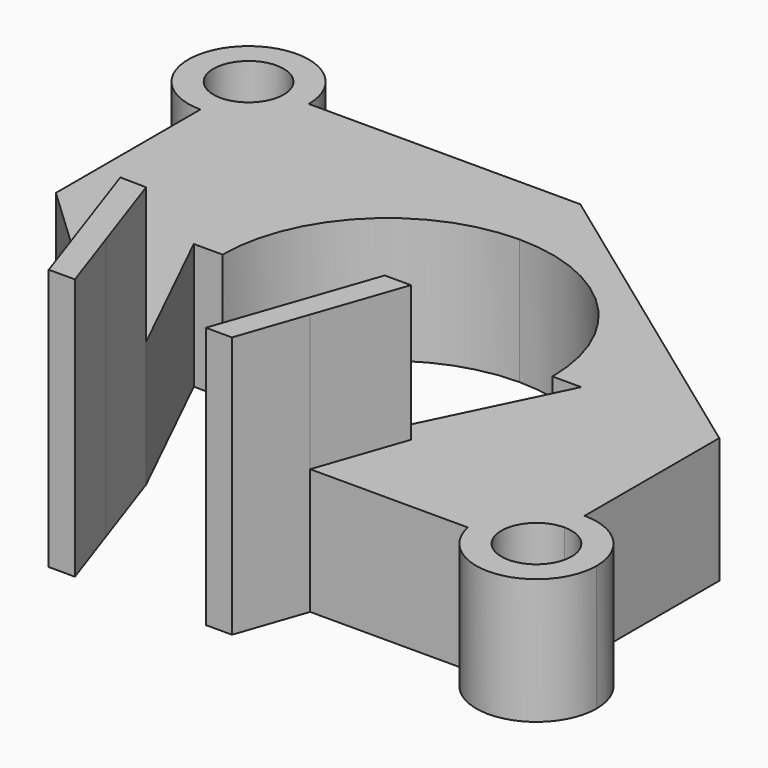
from build123d import *

# Parameters (mm, degrees)
F1_DEPTH = 12
F2_DEPTH = 25


# Not quite as in the source:
# - ends of sketch curves that miss each other by under 0.0002 mm in the source are joined


with BuildPart() as f1:
    # F0 (on Top) → F1 (new body)
    with BuildSketch(Plane.XY):
        with BuildLine():
            ThreePointArc((-55.8174114415, 34.8348648238), (-58.1862191586, 40.5536725408), (-52.4674114416, 38.1848648238))
            Line((-52.4674114416, 38.1848648238), (-50.0674114416, 38.1848649627))
            ThreePointArc((-50.0674114416, 38.1848649627), (-59.8832754334, 42.2507288156), (-55.8174114415, 32.4348648238))
            Line((-55.8174114415, 32.4348648238), (-55.8174114415, 34.8348648238))
        make_face()
        with BuildLine():
            Line((-50.0674114416, 38.1848649627), (-52.4674114416, 38.1848649047))
            ThreePointArc((-52.4674114416, 38.1848649047), (-53.4486037246, 35.8160571069), (-55.8174114415, 34.8348648238))
            Line((-55.8174114415, 34.8348648238), (-55.8174114415, 32.4348648238))
            ThreePointArc((-55.8174114415, 32.4348648238), (-51.7515474497, 34.119000832), (-50.0674114416, 38.1848649627))
        make_face()
        with BuildLine():
            Line((-24.1338443596, 38.184865589), (-50.0674114416, 38.1848649627))
            ThreePointArc((-50.0674114416, 38.1848649627), (-51.7515474497, 34.119000832), (-55.8174114415, 32.4348648238))
            Line((-55.8174114415, 32.4348648238), (-55.8174114412, 15.1848640586))
            Line((-55.8174114412, 15.1848640586), (-42.6338443592, 15.1659585535))
            ThreePointArc((-42.6338443592, 15.1659585535), (-37.2153198113, 28.2474340054), (-24.1338443595, 33.6659585535))
            Line((-24.1338443595, 33.6659585535), (-24.1338443596, 38.184865589))
        make_face()
        with BuildLine():
            Line((-24.1338443595, 30.9159585535), (-24.1338443595, 33.6659585535))
            ThreePointArc((-24.1338443595, 33.6659585535), (-37.2153198113, 28.2474340054), (-42.6338443592, 15.1659585535))
            Line((-42.6338443592, 15.1659585535), (-39.8838443592, 15.1659585535))
            ThreePointArc((-39.8838443592, 15.1659585535), (-35.270776163, 26.3028903571), (-24.1338443595, 30.9159585535))
        make_face()
        with BuildLine():
            Line((7.5497227227, 15.1659585535), (-24.1338443596, 38.184865589))
            Line((-24.1338443596, 38.184865589), (-24.1338443595, 33.6659585535))
            ThreePointArc((-24.1338443595, 33.6659585535), (-11.0523689074, 28.2474340056), (-5.6338443592, 15.1659585535))
            Line((-5.6338443592, 15.1659585535), (7.5497227227, 15.1659585535))
        make_face()
        with BuildLine():
            ThreePointArc((-5.6338443592, 15.1659585535), (-11.0523689074, 28.2474340056), (-24.1338443595, 33.6659585535))
            Line((-24.1338443595, 33.6659585535), (-24.1338443595, 30.9159585535))
            ThreePointArc((-24.1338443595, 30.9159585535), (-12.9969125556, 26.3028903573), (-8.3838443592, 15.1659585535))
            Line((-8.3838443592, 15.1659585535), (-5.6338443592, 15.1659585535))
        make_face()
        with BuildLine():
            Line((7.549722723, -0.909568585), (7.5497227227, 15.1659585535))
            Line((7.5497227227, 15.1659585535), (-5.6338443592, 15.1659585535))
            Line((-5.6338443592, 15.1659585535), (-12.7387191109, 0.5919707473))
            Line((-12.7387191109, 0.5919707473), (-10.2387191109, 0.5919707473))
            Line((-10.2387191109, 0.5919707473), (-13.136122196, -7.8151351762))
            Line((-13.136122196, -7.8151351762), (1.9170354556, -7.8151351762))
            ThreePointArc((1.9170354556, -7.8151351762), (3.0939956275, -3.0251503303), (7.549722723, -0.909568585))
        make_face()
        Polygon((-42.6338443592, 15.1659585535), (-55.8174114412, 15.1848640586), (-36.8837256357, -2.690086035), (-38.0284454354, 0.643162408), (-35.5289696075, 0.5919707473), align=None)
        with BuildLine():
            ThreePointArc((13.2997227231, -6.659568585), (11.6155867149, -2.5937045931), (7.549722723, -0.909568585))
            ThreePointArc((7.549722723, -0.909568585), (3.0939956275, -3.0251503303), (1.9170354556, -7.8151351762))
            ThreePointArc((1.9170354556, -7.8151351762), (8.1304757738, -12.3801652229), (13.2997227231, -6.659568585))
        make_face()
        with BuildLine():
            ThreePointArc((10.8997227231, -6.659568585), (5.1809150061, -9.028376302), (7.549722723, -3.309568585))
            ThreePointArc((7.549722723, -3.309568585), (9.91853044, -4.290760868), (10.8997227231, -6.659568585))
        make_face(mode=Mode.SUBTRACT)
        Polygon((-38.0284454354, 0.643162408), (-36.8837256357, -2.690086035), (-35.1236572441, -7.8151351762), (-32.6315665225, -7.8151351762), (-35.5289696075, 0.5919707473), align=None)
        Polygon((-32.6315665225, -7.8151351762), (-35.1236572441, -7.8151351762), (-32.8838443592, -14.3371266833), (-30.3838443592, -14.3371266833), align=None)
        Polygon((-13.136122196, -7.8151351762), (-15.636122196, -7.8151351762), (-17.8838443592, -14.3371266833), (-15.3838443592, -14.3371266833), align=None)
        Polygon((-10.2387191109, 0.5919707473), (-12.7387191109, 0.5919707473), (-15.636122196, -7.8151351762), (-13.136122196, -7.8151351762), align=None)
    extrude(amount=F1_DEPTH)

    # F0 (on Top) → F2 (join)
    with BuildSketch(Plane.XY):
        Polygon((-38.0284454354, 0.643162408), (-36.8837256357, -2.690086035), (-35.1236572441, -7.8151351762), (-32.6315665225, -7.8151351762), (-35.5289696075, 0.5919707473), align=None)
        Polygon((-32.6315665225, -7.8151351762), (-35.1236572441, -7.8151351762), (-32.8838443592, -14.3371266833), (-30.3838443592, -14.3371266833), align=None)
        Polygon((-10.2387191109, 0.5919707473), (-12.7387191109, 0.5919707473), (-15.636122196, -7.8151351762), (-13.136122196, -7.8151351762), align=None)
        Polygon((-13.136122196, -7.8151351762), (-15.636122196, -7.8151351762), (-17.8838443592, -14.3371266833), (-15.3838443592, -14.3371266833), align=None)
    extrude(amount=F2_DEPTH)


solid = f1.part
